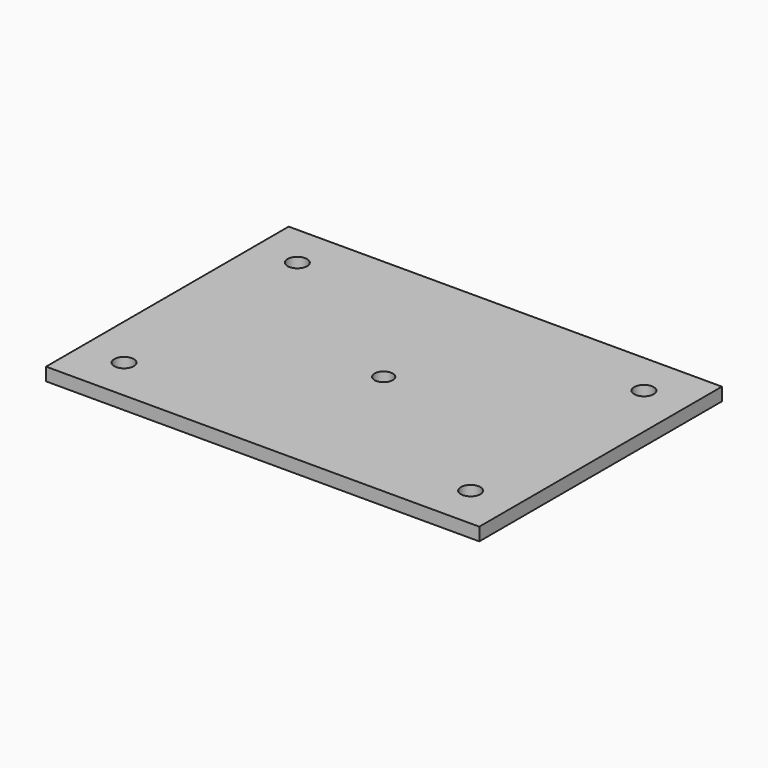
from build123d import *

# Parameters (mm, degrees)
F0_W     = 100
F0_H     = 70
F0_R     = 2.25
F0_R_2   = 2.1
F1_DEPTH = 3


# Not quite as in the source:
# - a feature names something its author has since deleted; it is built from what else it names


with BuildPart() as f1:
    # F0 (on Top) → F1 (new body)
    with BuildSketch(Plane.XY):
        with Locations((-7.451e-07, 0.0999978185)):
            Rectangle(F0_W, F0_H)
        with Locations((-40.0000007451, -24.9000021815)):
            Circle(F0_R, mode=Mode.SUBTRACT)
        with Locations((40.0000007451, -24.9000021815)):
            Circle(F0_R, mode=Mode.SUBTRACT)
        Circle(F0_R_2, mode=Mode.SUBTRACT)
        with Locations((-40.0000007451, 25.0999978185)):
            Circle(F0_R, mode=Mode.SUBTRACT)
        with Locations((40.0000007451, 25.0999978185)):
            Circle(F0_R, mode=Mode.SUBTRACT)
    extrude(amount=F1_DEPTH)


solid = f1.part
